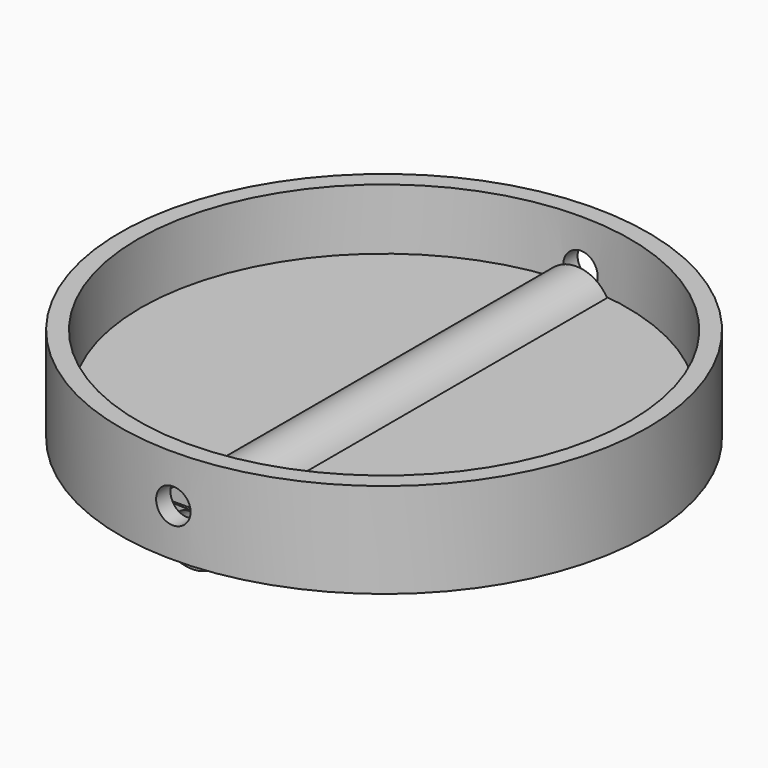
from build123d import *

# Parameters (mm, degrees)
F0_R          = 22.225
F0_R_2        = 20.725
F1_DEPTH      = 8
F0_R_3        = 20.475
F2_DEPTH      = 3
F3_R          = 3
F4_DEPTH      = 20.225
F4_DEPTH_BACK = 20.225
F5_R          = 1.45
F6_DEPTH      = 22.226
F6_DEPTH_BACK = 22.226
F7_R          = 1.4
F8_DEPTH      = 22.2260001181
F8_DEPTH_BACK = 22.2260001181


with BuildPart() as f1:
    # F0 (on Top) → F1 (new body)
    with BuildSketch(Plane.XY):
        Circle(F0_R)
        Circle(F0_R_2, mode=Mode.SUBTRACT)
    extrude(amount=F1_DEPTH)

    # F5 (on Front) → F6 (cut, two sides)
    with BuildSketch(Plane.XZ) as f6_sk:
        with Locations((0, 4)):
            Circle(F5_R)
    extrude(amount=-F6_DEPTH, mode=Mode.SUBTRACT)
    extrude(f6_sk.sketch, amount=F6_DEPTH_BACK, mode=Mode.SUBTRACT)


with BuildPart() as f2:
    # F0 (on Top) → F2 (new body)
    with BuildSketch(Plane.XY):
        Circle(F0_R_3)
    extrude(amount=F2_DEPTH)

    # F3 (on Front) → F4 (join, two sides)
    with BuildSketch(Plane.XZ) as f4_sk:
        with Locations((0, 1.5)):
            Circle(F3_R)
    extrude(amount=F4_DEPTH)
    extrude(f4_sk.sketch, amount=-F4_DEPTH_BACK)

    # F7 (on Front) → F8 (cut, two sides)
    with BuildSketch(Plane.XZ) as f8_sk:
        with Locations((0, 1.5)):
            Circle(F7_R)
    extrude(amount=-F8_DEPTH, mode=Mode.SUBTRACT)
    extrude(f8_sk.sketch, amount=F8_DEPTH_BACK, mode=Mode.SUBTRACT)


solid = Compound([f1.part, f2.part])
